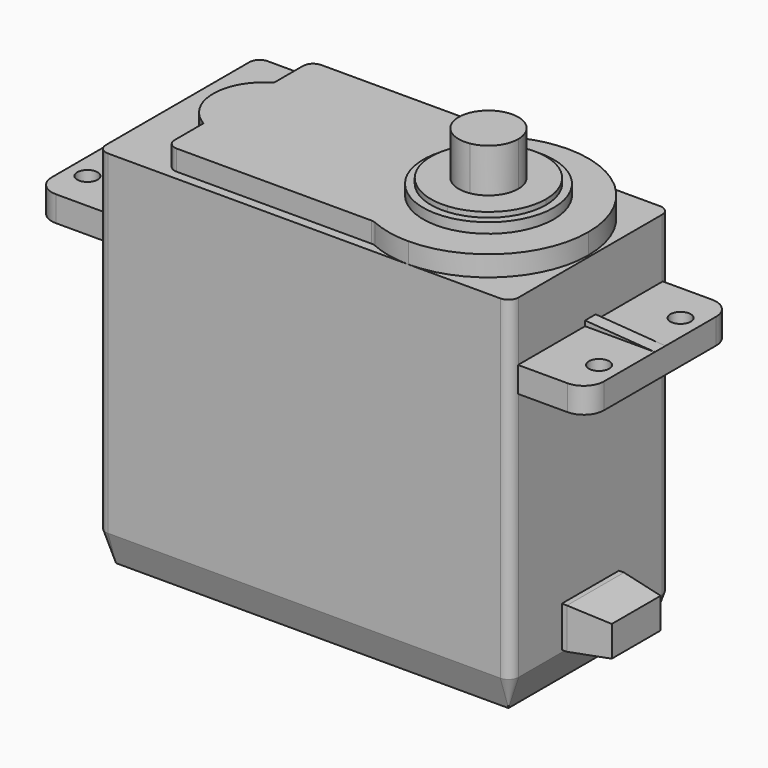
from build123d import *

# Parameters (mm, degrees)
F0_W           = 40.5
F0_H           = 2.5
F1_DEPTH       = 9.8
F0_W_2         = 6.85
F2_DEPTH       = 8.875
F0_W_3         = 4.5
F0_H_2         = 4
F3_DEPTH       = 3.5
F4_SIZE2       = 0.5
F4_SIZE        = 4
F6_DEPTH       = 2
F7_DEPTH       = 3
F8_DEPTH       = 3.5
F9_DEPTH       = 7.8
F10_DEPTH      = 0.65
F11_R          = 1
F12_DEPTH      = 5
F13_R          = 2
F14_R          = 1
F15_T4_DEPTH   = 40.8
F15_T10_DEPTH  = 40.8
F15_T16_DEPTH  = 40.8
F15_T23_DEPTH  = 40.8
F15_T29_DEPTH  = 40.8
F15_T35_DEPTH  = 40.8
F15_T41_DEPTH  = 40.8
F15_T47_DEPTH  = 40.8
F15_T54_DEPTH  = 40.8
F15_T60_DEPTH  = 40.8
F15_T66_DEPTH  = 40.8
F15_T72_DEPTH  = 40.8
F15_T78_DEPTH  = 40.8
F15_T85_DEPTH  = 40.8
F15_T91_DEPTH  = 40.8
F15_T97_DEPTH  = 40.8
F15_T103_DEPTH = 40.8
F15_T109_DEPTH = 40.8
F15_T116_DEPTH = 40.8
F15_T122_DEPTH = 40.8
F16_T1_DEPTH   = 38.5
F16_T3_DEPTH   = 17.6
F16_T6_ANGLE   = 90.0000000053
F16_T8_ANGLE   = 90.0000000053
F16_T10_ANGLE  = 90.0000000053
F16_T12_ANGLE  = 90.0000000053


# Not quite as in the source:
# - a fillet or chamfer that OpenCascade refuses, or shapes differently, is made with other operations: its cross-section is extruded or revolved along the edge and cut away or added


with BuildPart() as f1:
    # F0 (on Front) → F1 (new body, symmetric)
    with BuildSketch(Plane.XZ):
        Polygon((20.25, 17.9), (-20.25, 17.9), (-20.25, 12.6), (-20.25, 12.1), (20.25, 12.1), (20.25, 12.6), align=None)
        Polygon((20.25, 9.6), (-20.25, 9.6), (-20.25, -17.9), (20.25, -17.9), (20.25, -14.7), (20.25, -10.7), align=None)
        with Locations((0, 10.85)):
            Rectangle(F0_W, F0_H)
    extrude(amount=F1_DEPTH, both=True)

    # F0 (on Front) → F2 (join, symmetric)
    with BuildSketch(Plane.XZ):
        with Locations((23.675, 10.85)):
            Rectangle(F0_W_2, F0_H)
        with Locations((-23.675, 10.85)):
            Rectangle(F0_W_2, F0_H)
    extrude(amount=F2_DEPTH, both=True)

    # F0 (on Front) → F3 (join, symmetric)
    with BuildSketch(Plane.XZ):
        with Locations((22.5, -12.7)):
            Rectangle(F0_W_3, F0_H_2)
    extrude(amount=F3_DEPTH, both=True)

    # F4
    f4_edges = [f1.edges().sort_by_distance(p)[0] for p in [
        (24.75, 0, -10.7),
        (24.75, 3.5, -12.7),
        (24.75, -3.5, -12.7),
        (24.75, 0, -14.7),
    ]]
    chamfer(f4_edges, length=F4_SIZE, length2=F4_SIZE2)

    # F5 (on face) → F6 (join)
    with BuildSketch(Plane.XY.offset(17.9)):
        with BuildLine():
            ThreePointArc((10.2500000427, -9.8), (17.1796464707, -6.9296464405), (20.05, 0))
            ThreePointArc((20.05, 0), (17.1796464556, 6.9296464556), (10.25, 9.8))
            ThreePointArc((10.25, 9.8), (8.1210331144, 9.5659552581), (6.0937546993, 8.875))
            Line((6.0937546993, 8.875), (10.75, 8.875))
            Line((10.75, 8.875), (10.75, 6.3804388564))
            ThreePointArc((10.75, 6.3804388564), (14.9489360498, 4.3451121965), (16.65, 0))
            ThreePointArc((16.65, 0), (14.9489360498, -4.3451121965), (10.75, -6.3804388564))
            Line((10.75, -6.3804388564), (10.75, -8.875))
            Line((10.75, -8.875), (6.0937546993, -8.875))
            ThreePointArc((6.0937546993, -8.875), (8.1210331353, -9.5659552627), (10.2500000427, -9.8))
        make_face()
        with BuildLine():
            ThreePointArc((16.65, 0), (14.9489360498, 4.3451121965), (10.75, 6.3804388564))
            Line((10.75, 6.3804388564), (10.75, 5.6278326201))
            ThreePointArc((10.75, 5.6278326201), (14.4181830574, 3.8142823702), (15.9, 0))
            ThreePointArc((15.9, 0), (14.4181830574, -3.8142823702), (10.75, -5.6278326201))
            Line((10.75, -5.6278326201), (10.75, -6.3804388564))
            ThreePointArc((10.75, -6.3804388564), (14.9489360498, -4.3451121965), (16.65, 0))
        make_face()
        with BuildLine():
            ThreePointArc((15.9, 0), (14.4181830574, 3.8142823702), (10.75, 5.6278326201))
            Line((10.75, 5.6278326201), (10.75, 2.8819481258))
            ThreePointArc((10.75, 2.8819481258), (12.4880934967, 1.8832319294), (13.175, 0))
            ThreePointArc((13.175, 0), (12.4880934967, -1.8832319294), (10.75, -2.8819481258))
            Line((10.75, -2.8819481258), (10.75, -5.6278326201))
            ThreePointArc((10.75, -5.6278326201), (14.4181830574, -3.8142823702), (15.9, 0))
        make_face()
        with BuildLine():
            Line((10.75, 2.8819481258), (10.75, 5.6278326201))
            ThreePointArc((10.75, 5.6278326201), (4.6, 0), (10.75, -5.6278326201))
            Line((10.75, -5.6278326201), (10.75, -2.8819481258))
            ThreePointArc((10.75, -2.8819481258), (7.325, 0), (10.75, 2.8819481258))
        make_face()
        with BuildLine():
            Line((10.75, -2.8819481258), (10.75, 2.8819481258))
            ThreePointArc((10.75, 2.8819481258), (7.325, 0), (10.75, -2.8819481258))
        make_face()
        with BuildLine():
            ThreePointArc((13.175, 0), (12.4880934967, 1.8832319294), (10.75, 2.8819481258))
            Line((10.75, 2.8819481258), (10.75, -2.8819481258))
            ThreePointArc((10.75, -2.8819481258), (12.4880934967, -1.8832319294), (13.175, 0))
        make_face()
        with BuildLine():
            Line((10.75, 5.6278326201), (10.75, 6.3804388564))
            ThreePointArc((10.75, 6.3804388564), (3.85, 0), (10.75, -6.3804388564))
            Line((10.75, -6.3804388564), (10.75, -5.6278326201))
            ThreePointArc((10.75, -5.6278326201), (4.6, 0), (10.75, 5.6278326201))
        make_face()
        with BuildLine():
            Line((10.75, 8.875), (6.0937546993, 8.875))
            ThreePointArc((6.0937546993, 8.875), (0.45, 0), (6.0937546993, -8.875))
            Line((6.0937546993, -8.875), (10.75, -8.875))
            Line((10.75, -8.875), (10.75, -6.3804388564))
            ThreePointArc((10.75, -6.3804388564), (3.85, 0), (10.75, 6.3804388564))
            Line((10.75, 6.3804388564), (10.75, 8.875))
        make_face()
        with BuildLine():
            ThreePointArc((6.0937546993, -8.875), (0.45, 0), (6.0937546993, 8.875))
            Line((6.0937546993, 8.875), (-14.25, 8.875))
            Line((-14.25, 8.875), (-14.25, 4.3301270189))
            ThreePointArc((-14.25, 4.3301270189), (-9.25, 4.3301270189), (-6.75, 0))
            ThreePointArc((-6.75, 0), (-9.25, -4.3301270189), (-14.25, -4.3301270189))
            Line((-14.25, -4.3301270189), (-14.25, -8.875))
            Line((-14.25, -8.875), (6.0937546993, -8.875))
        make_face()
        with BuildLine():
            ThreePointArc((-6.75, 0), (-9.25, 4.3301270189), (-14.25, 4.3301270189))
            Line((-14.25, 4.3301270189), (-14.25, -4.3301270189))
            ThreePointArc((-14.25, -4.3301270189), (-9.25, -4.3301270189), (-6.75, 0))
        make_face()
        with BuildLine():
            Line((-14.25, -4.3301270189), (-14.25, 4.3301270189))
            ThreePointArc((-14.25, 4.3301270189), (-16.75, 0), (-14.25, -4.3301270189))
        make_face()
    extrude(amount=F6_DEPTH)

    # F5 (on face) → F7 (join)
    with BuildSketch(Plane.XY.offset(17.9)):
        with BuildLine():
            Line((10.75, 2.8819481258), (10.75, 5.6278326201))
            ThreePointArc((10.75, 5.6278326201), (4.6, 0), (10.75, -5.6278326201))
            Line((10.75, -5.6278326201), (10.75, -2.8819481258))
            ThreePointArc((10.75, -2.8819481258), (7.325, 0), (10.75, 2.8819481258))
        make_face()
        with BuildLine():
            Line((10.75, -2.8819481258), (10.75, 2.8819481258))
            ThreePointArc((10.75, 2.8819481258), (7.325, 0), (10.75, -2.8819481258))
        make_face()
        with BuildLine():
            ThreePointArc((13.175, 0), (12.4880934967, 1.8832319294), (10.75, 2.8819481258))
            Line((10.75, 2.8819481258), (10.75, -2.8819481258))
            ThreePointArc((10.75, -2.8819481258), (12.4880934967, -1.8832319294), (13.175, 0))
        make_face()
        with BuildLine():
            ThreePointArc((15.9, 0), (14.4181830574, 3.8142823702), (10.75, 5.6278326201))
            Line((10.75, 5.6278326201), (10.75, 2.8819481258))
            ThreePointArc((10.75, 2.8819481258), (12.4880934967, 1.8832319294), (13.175, 0))
            ThreePointArc((13.175, 0), (12.4880934967, -1.8832319294), (10.75, -2.8819481258))
            Line((10.75, -2.8819481258), (10.75, -5.6278326201))
            ThreePointArc((10.75, -5.6278326201), (14.4181830574, -3.8142823702), (15.9, 0))
        make_face()
        with BuildLine():
            ThreePointArc((16.65, 0), (14.9489360498, 4.3451121965), (10.75, 6.3804388564))
            Line((10.75, 6.3804388564), (10.75, 5.6278326201))
            ThreePointArc((10.75, 5.6278326201), (14.4181830574, 3.8142823702), (15.9, 0))
            ThreePointArc((15.9, 0), (14.4181830574, -3.8142823702), (10.75, -5.6278326201))
            Line((10.75, -5.6278326201), (10.75, -6.3804388564))
            ThreePointArc((10.75, -6.3804388564), (14.9489360498, -4.3451121965), (16.65, 0))
        make_face()
        with BuildLine():
            Line((10.75, 5.6278326201), (10.75, 6.3804388564))
            ThreePointArc((10.75, 6.3804388564), (3.85, 0), (10.75, -6.3804388564))
            Line((10.75, -6.3804388564), (10.75, -5.6278326201))
            ThreePointArc((10.75, -5.6278326201), (4.6, 0), (10.75, 5.6278326201))
        make_face()
    extrude(amount=F7_DEPTH)

    # F5 (on face) → F8 (join)
    with BuildSketch(Plane.XY.offset(17.9)):
        with BuildLine():
            ThreePointArc((13.175, 0), (12.4880934967, 1.8832319294), (10.75, 2.8819481258))
            Line((10.75, 2.8819481258), (10.75, -2.8819481258))
            ThreePointArc((10.75, -2.8819481258), (12.4880934967, -1.8832319294), (13.175, 0))
        make_face()
        with BuildLine():
            Line((10.75, -2.8819481258), (10.75, 2.8819481258))
            ThreePointArc((10.75, 2.8819481258), (7.325, 0), (10.75, -2.8819481258))
        make_face()
        with BuildLine():
            Line((10.75, 2.8819481258), (10.75, 5.6278326201))
            ThreePointArc((10.75, 5.6278326201), (4.6, 0), (10.75, -5.6278326201))
            Line((10.75, -5.6278326201), (10.75, -2.8819481258))
            ThreePointArc((10.75, -2.8819481258), (7.325, 0), (10.75, 2.8819481258))
        make_face()
        with BuildLine():
            ThreePointArc((15.9, 0), (14.4181830574, 3.8142823702), (10.75, 5.6278326201))
            Line((10.75, 5.6278326201), (10.75, 2.8819481258))
            ThreePointArc((10.75, 2.8819481258), (12.4880934967, 1.8832319294), (13.175, 0))
            ThreePointArc((13.175, 0), (12.4880934967, -1.8832319294), (10.75, -2.8819481258))
            Line((10.75, -2.8819481258), (10.75, -5.6278326201))
            ThreePointArc((10.75, -5.6278326201), (14.4181830574, -3.8142823702), (15.9, 0))
        make_face()
    extrude(amount=F8_DEPTH)

    # F5 (on face) → F9 (join)
    with BuildSketch(Plane.XY.offset(17.9)):
        with BuildLine():
            Line((10.75, -2.8819481258), (10.75, 2.8819481258))
            ThreePointArc((10.75, 2.8819481258), (7.325, 0), (10.75, -2.8819481258))
        make_face()
        with BuildLine():
            ThreePointArc((13.175, 0), (12.4880934967, 1.8832319294), (10.75, 2.8819481258))
            Line((10.75, 2.8819481258), (10.75, -2.8819481258))
            ThreePointArc((10.75, -2.8819481258), (12.4880934967, -1.8832319294), (13.175, 0))
        make_face()
    extrude(amount=F9_DEPTH)

    # F0 (on Front) → F10 (join, symmetric)
    with BuildSketch(Plane.XZ):
        Polygon((27.1, 12.1), (20.25, 12.6), (20.25, 12.1), align=None)
        Polygon((-20.25, 12.1), (-20.25, 12.6), (-27.1, 12.1), align=None)
    extrude(amount=F10_DEPTH, both=True)

    # F11 (on face) → F12 (cut)
    with BuildSketch(Plane.XY.offset(12.1)):
        with Locations((-25.1, 5)):
            Circle(F11_R)
        with Locations((-25.1, -5)):
            Circle(F11_R)
        with Locations((25.1, 5)):
            Circle(F11_R)
        with Locations((25.1, -5)):
            Circle(F11_R)
    extrude(amount=-F12_DEPTH, mode=Mode.SUBTRACT)

    # F13
    f13_edges = [f1.edges().sort_by_distance(p)[0] for p in [
        (27.1, -8.875, 10.85),
        (27.1, 8.875, 10.85),
        (-27.1, -8.875, 10.85),
        (-27.1, 8.875, 10.85),
    ]]
    fillet(f13_edges, radius=F13_R)

    # F14
    f14_edges = [f1.edges().sort_by_distance(p)[0] for p in [
        (-14.25, -8.875, 18.9),
        (-14.25, 8.875, 18.9),
        (6.093755, 8.875, 18.9),
        (6.093755, -8.875, 18.9),
    ]]
    fillet(f14_edges, radius=F14_R)

    # F15: fillet of radius 1 on 4 edges, made by hand


with BuildPart() as f15_tool2:
    # F15_s3 → F15_t4 (new body)
    with BuildSketch(Plane.XY.offset(-20.4)):
        with BuildLine():
            ThreePointArc((19.25, -9.8), (19.9571067812, -9.5071067812), (20.25, -8.8))
            Line((20.25, -8.8), (20.25, -9.8))
            Line((20.25, -9.8), (19.25, -9.8))
        make_face()
    extrude(amount=F15_T4_DEPTH)

    split(bisect_by=Plane.XZ.offset(8.875), keep=Keep.TOP)

    split(bisect_by=Plane.XY.offset(9.6), keep=Keep.BOTTOM)


with BuildPart() as f1_1:
    add(f1.part)

    # F15_t1: cut F15_tool2
    add(f15_tool2.part, mode=Mode.SUBTRACT)


with BuildPart() as f15_tool8:
    # F15_s9 → F15_t10 (new body)
    with BuildSketch(Plane.XY.offset(-20.4)):
        with BuildLine():
            ThreePointArc((19.25, -9.8), (19.9571067812, -9.5071067812), (20.25, -8.8))
            Line((20.25, -8.8), (20.25, -9.8))
            Line((20.25, -9.8), (19.25, -9.8))
        make_face()
    extrude(amount=F15_T10_DEPTH)

    split(bisect_by=Plane.XZ.offset(8.875), keep=Keep.BOTTOM)

    split(bisect_by=Plane.XY.offset(9.6), keep=Keep.BOTTOM)


with BuildPart() as f1_2:
    add(f1_1.part)

    # F15_t7: cut F15_tool8
    add(f15_tool8.part, mode=Mode.SUBTRACT)


with BuildPart() as f15_tool14:
    # F15_s15 → F15_t16 (new body)
    with BuildSketch(Plane.XY.offset(-20.4)):
        with BuildLine():
            ThreePointArc((19.25, -9.8), (19.9571067812, -9.5071067812), (20.25, -8.8))
            Line((20.25, -8.8), (20.25, -9.8))
            Line((20.25, -9.8), (19.25, -9.8))
        make_face()
    extrude(amount=F15_T16_DEPTH)

    split(bisect_by=Plane.XY.offset(12.1), keep=Keep.BOTTOM)

    split(bisect_by=Plane.XZ.offset(8.875), keep=Keep.TOP)

    split(bisect_by=Plane.XY.offset(9.6), keep=Keep.TOP)


with BuildPart() as f1_3:
    add(f1_2.part)

    # F15_t13: cut F15_tool14
    add(f15_tool14.part, mode=Mode.SUBTRACT)


with BuildPart() as f15_tool21:
    # F15_s22 → F15_t23 (new body)
    with BuildSketch(Plane.XY.offset(-20.4)):
        with BuildLine():
            ThreePointArc((19.25, -9.8), (19.9571067812, -9.5071067812), (20.25, -8.8))
            Line((20.25, -8.8), (20.25, -9.8))
            Line((20.25, -9.8), (19.25, -9.8))
        make_face()
    extrude(amount=F15_T23_DEPTH)

    split(bisect_by=Plane.XY.offset(12.1), keep=Keep.TOP)

    split(bisect_by=Plane.XZ.offset(8.875), keep=Keep.TOP)


with BuildPart() as f1_4:
    add(f1_3.part)

    # F15_t20: cut F15_tool21
    add(f15_tool21.part, mode=Mode.SUBTRACT)


with BuildPart() as f15_tool27:
    # F15_s28 → F15_t29 (new body)
    with BuildSketch(Plane.XY.offset(-20.4)):
        with BuildLine():
            ThreePointArc((19.25, -9.8), (19.9571067812, -9.5071067812), (20.25, -8.8))
            Line((20.25, -8.8), (20.25, -9.8))
            Line((20.25, -9.8), (19.25, -9.8))
        make_face()
    extrude(amount=F15_T29_DEPTH)

    split(bisect_by=Plane.XY.offset(12.1), keep=Keep.TOP)

    split(bisect_by=Plane.XZ.offset(8.875), keep=Keep.BOTTOM)


with BuildPart() as f1_5:
    add(f1_4.part)

    # F15_t26: cut F15_tool27
    add(f15_tool27.part, mode=Mode.SUBTRACT)


with BuildPart() as f15_tool33:
    # F15_s34 → F15_t35 (new body)
    with BuildSketch(Plane.XY.offset(20.4)):
        with BuildLine():
            ThreePointArc((-20.25, -8.8), (-19.9571067812, -9.5071067812), (-19.25, -9.8))
            Line((-19.25, -9.8), (-20.25, -9.8))
            Line((-20.25, -9.8), (-20.25, -8.8))
        make_face()
    extrude(amount=-F15_T35_DEPTH)

    split(bisect_by=Plane.XZ.offset(8.875), keep=Keep.BOTTOM)

    split(bisect_by=Plane.XY.offset(12.1), keep=Keep.TOP)


with BuildPart() as f1_6:
    add(f1_5.part)

    # F15_t32: cut F15_tool33
    add(f15_tool33.part, mode=Mode.SUBTRACT)


with BuildPart() as f15_tool39:
    # F15_s40 → F15_t41 (new body)
    with BuildSketch(Plane.XY.offset(20.4)):
        with BuildLine():
            ThreePointArc((-20.25, -8.8), (-19.9571067812, -9.5071067812), (-19.25, -9.8))
            Line((-19.25, -9.8), (-20.25, -9.8))
            Line((-20.25, -9.8), (-20.25, -8.8))
        make_face()
    extrude(amount=-F15_T41_DEPTH)

    split(bisect_by=Plane.XZ.offset(8.875), keep=Keep.TOP)

    split(bisect_by=Plane.XY.offset(12.1), keep=Keep.TOP)


with BuildPart() as f1_7:
    add(f1_6.part)

    # F15_t38: cut F15_tool39
    add(f15_tool39.part, mode=Mode.SUBTRACT)


with BuildPart() as f15_tool45:
    # F15_s46 → F15_t47 (new body)
    with BuildSketch(Plane.XY.offset(20.4)):
        with BuildLine():
            ThreePointArc((-20.25, -8.8), (-19.9571067812, -9.5071067812), (-19.25, -9.8))
            Line((-19.25, -9.8), (-20.25, -9.8))
            Line((-20.25, -9.8), (-20.25, -8.8))
        make_face()
    extrude(amount=-F15_T47_DEPTH)

    split(bisect_by=Plane.XZ.offset(8.875), keep=Keep.TOP)

    split(bisect_by=Plane.XY.offset(12.1), keep=Keep.BOTTOM)

    split(bisect_by=Plane.XY.offset(9.6), keep=Keep.TOP)


with BuildPart() as f1_8:
    add(f1_7.part)

    # F15_t44: cut F15_tool45
    add(f15_tool45.part, mode=Mode.SUBTRACT)


with BuildPart() as f15_tool52:
    # F15_s53 → F15_t54 (new body)
    with BuildSketch(Plane.XY.offset(20.4)):
        with BuildLine():
            ThreePointArc((-20.25, -8.8), (-19.9571067812, -9.5071067812), (-19.25, -9.8))
            Line((-19.25, -9.8), (-20.25, -9.8))
            Line((-20.25, -9.8), (-20.25, -8.8))
        make_face()
    extrude(amount=-F15_T54_DEPTH)

    split(bisect_by=Plane.XZ.offset(8.875), keep=Keep.BOTTOM)

    split(bisect_by=Plane.XY.offset(9.6), keep=Keep.BOTTOM)


with BuildPart() as f1_9:
    add(f1_8.part)

    # F15_t51: cut F15_tool52
    add(f15_tool52.part, mode=Mode.SUBTRACT)


with BuildPart() as f15_tool58:
    # F15_s59 → F15_t60 (new body)
    with BuildSketch(Plane.XY.offset(20.4)):
        with BuildLine():
            ThreePointArc((-20.25, -8.8), (-19.9571067812, -9.5071067812), (-19.25, -9.8))
            Line((-19.25, -9.8), (-20.25, -9.8))
            Line((-20.25, -9.8), (-20.25, -8.8))
        make_face()
    extrude(amount=-F15_T60_DEPTH)

    split(bisect_by=Plane.XZ.offset(8.875), keep=Keep.TOP)

    split(bisect_by=Plane.XY.offset(9.6), keep=Keep.BOTTOM)


with BuildPart() as f1_10:
    add(f1_9.part)

    # F15_t57: cut F15_tool58
    add(f15_tool58.part, mode=Mode.SUBTRACT)


with BuildPart() as f15_tool64:
    # F15_s65 → F15_t66 (new body)
    with BuildSketch(Plane.XY.offset(20.4)):
        with BuildLine():
            ThreePointArc((-19.25, 9.8), (-19.9571067812, 9.5071067812), (-20.25, 8.8))
            Line((-20.25, 8.8), (-20.25, 9.8))
            Line((-20.25, 9.8), (-19.25, 9.8))
        make_face()
    extrude(amount=-F15_T66_DEPTH)

    split(bisect_by=Plane.XY.offset(12.1), keep=Keep.TOP)

    split(bisect_by=Plane.XZ.offset(-8.875), keep=Keep.BOTTOM)


with BuildPart() as f1_11:
    add(f1_10.part)

    # F15_t63: cut F15_tool64
    add(f15_tool64.part, mode=Mode.SUBTRACT)


with BuildPart() as f15_tool70:
    # F15_s71 → F15_t72 (new body)
    with BuildSketch(Plane.XY.offset(20.4)):
        with BuildLine():
            ThreePointArc((-19.25, 9.8), (-19.9571067812, 9.5071067812), (-20.25, 8.8))
            Line((-20.25, 8.8), (-20.25, 9.8))
            Line((-20.25, 9.8), (-19.25, 9.8))
        make_face()
    extrude(amount=-F15_T72_DEPTH)

    split(bisect_by=Plane.XY.offset(12.1), keep=Keep.TOP)

    split(bisect_by=Plane.XZ.offset(-8.875), keep=Keep.TOP)


with BuildPart() as f1_12:
    add(f1_11.part)

    # F15_t69: cut F15_tool70
    add(f15_tool70.part, mode=Mode.SUBTRACT)


with BuildPart() as f15_tool76:
    # F15_s77 → F15_t78 (new body)
    with BuildSketch(Plane.XY.offset(20.4)):
        with BuildLine():
            ThreePointArc((-19.25, 9.8), (-19.9571067812, 9.5071067812), (-20.25, 8.8))
            Line((-20.25, 8.8), (-20.25, 9.8))
            Line((-20.25, 9.8), (-19.25, 9.8))
        make_face()
    extrude(amount=-F15_T78_DEPTH)

    split(bisect_by=Plane.XY.offset(12.1), keep=Keep.BOTTOM)

    split(bisect_by=Plane.XZ.offset(-8.875), keep=Keep.BOTTOM)

    split(bisect_by=Plane.XY.offset(9.6), keep=Keep.TOP)


with BuildPart() as f1_13:
    add(f1_12.part)

    # F15_t75: cut F15_tool76
    add(f15_tool76.part, mode=Mode.SUBTRACT)


with BuildPart() as f15_tool83:
    # F15_s84 → F15_t85 (new body)
    with BuildSketch(Plane.XY.offset(20.4)):
        with BuildLine():
            ThreePointArc((-19.25, 9.8), (-19.9571067812, 9.5071067812), (-20.25, 8.8))
            Line((-20.25, 8.8), (-20.25, 9.8))
            Line((-20.25, 9.8), (-19.25, 9.8))
        make_face()
    extrude(amount=-F15_T85_DEPTH)

    split(bisect_by=Plane.XZ.offset(-8.875), keep=Keep.BOTTOM)

    split(bisect_by=Plane.XY.offset(9.6), keep=Keep.BOTTOM)


with BuildPart() as f1_14:
    add(f1_13.part)

    # F15_t82: cut F15_tool83
    add(f15_tool83.part, mode=Mode.SUBTRACT)


with BuildPart() as f15_tool89:
    # F15_s90 → F15_t91 (new body)
    with BuildSketch(Plane.XY.offset(20.4)):
        with BuildLine():
            ThreePointArc((-19.25, 9.8), (-19.9571067812, 9.5071067812), (-20.25, 8.8))
            Line((-20.25, 8.8), (-20.25, 9.8))
            Line((-20.25, 9.8), (-19.25, 9.8))
        make_face()
    extrude(amount=-F15_T91_DEPTH)

    split(bisect_by=Plane.XZ.offset(-8.875), keep=Keep.TOP)

    split(bisect_by=Plane.XY.offset(9.6), keep=Keep.BOTTOM)


with BuildPart() as f1_15:
    add(f1_14.part)

    # F15_t88: cut F15_tool89
    add(f15_tool89.part, mode=Mode.SUBTRACT)


with BuildPart() as f15_tool95:
    # F15_s96 → F15_t97 (new body)
    with BuildSketch(Plane.XY.offset(-20.4)):
        with BuildLine():
            ThreePointArc((19.25, 9.8), (19.9571067812, 9.5071067812), (20.25, 8.8))
            Line((20.25, 8.8), (20.25, 9.8))
            Line((20.25, 9.8), (19.25, 9.8))
        make_face()
    extrude(amount=F15_T97_DEPTH)

    split(bisect_by=Plane.XY.offset(9.6), keep=Keep.BOTTOM)

    split(bisect_by=Plane.XZ.offset(-8.875), keep=Keep.BOTTOM)


with BuildPart() as f1_16:
    add(f1_15.part)

    # F15_t94: cut F15_tool95
    add(f15_tool95.part, mode=Mode.SUBTRACT)


with BuildPart() as f15_tool101:
    # F15_s102 → F15_t103 (new body)
    with BuildSketch(Plane.XY.offset(-20.4)):
        with BuildLine():
            ThreePointArc((19.25, 9.8), (19.9571067812, 9.5071067812), (20.25, 8.8))
            Line((20.25, 8.8), (20.25, 9.8))
            Line((20.25, 9.8), (19.25, 9.8))
        make_face()
    extrude(amount=F15_T103_DEPTH)

    split(bisect_by=Plane.XY.offset(9.6), keep=Keep.BOTTOM)

    split(bisect_by=Plane.XZ.offset(-8.875), keep=Keep.TOP)


with BuildPart() as f1_17:
    add(f1_16.part)

    # F15_t100: cut F15_tool101
    add(f15_tool101.part, mode=Mode.SUBTRACT)


with BuildPart() as f15_tool107:
    # F15_s108 → F15_t109 (new body)
    with BuildSketch(Plane.XY.offset(-20.4)):
        with BuildLine():
            ThreePointArc((19.25, 9.8), (19.9571067812, 9.5071067812), (20.25, 8.8))
            Line((20.25, 8.8), (20.25, 9.8))
            Line((20.25, 9.8), (19.25, 9.8))
        make_face()
    extrude(amount=F15_T109_DEPTH)

    split(bisect_by=Plane.XY.offset(12.1), keep=Keep.BOTTOM)

    split(bisect_by=Plane.XY.offset(9.6), keep=Keep.TOP)

    split(bisect_by=Plane.XZ.offset(-8.875), keep=Keep.BOTTOM)


with BuildPart() as f1_18:
    add(f1_17.part)

    # F15_t106: cut F15_tool107
    add(f15_tool107.part, mode=Mode.SUBTRACT)


with BuildPart() as f15_tool114:
    # F15_s115 → F15_t116 (new body)
    with BuildSketch(Plane.XY.offset(-20.4)):
        with BuildLine():
            ThreePointArc((19.25, 9.8), (19.9571067812, 9.5071067812), (20.25, 8.8))
            Line((20.25, 8.8), (20.25, 9.8))
            Line((20.25, 9.8), (19.25, 9.8))
        make_face()
    extrude(amount=F15_T116_DEPTH)

    split(bisect_by=Plane.XY.offset(12.1), keep=Keep.TOP)

    split(bisect_by=Plane.XZ.offset(-8.875), keep=Keep.BOTTOM)


with BuildPart() as f1_19:
    add(f1_18.part)

    # F15_t113: cut F15_tool114
    add(f15_tool114.part, mode=Mode.SUBTRACT)


with BuildPart() as f15_tool120:
    # F15_s121 → F15_t122 (new body)
    with BuildSketch(Plane.XY.offset(-20.4)):
        with BuildLine():
            ThreePointArc((19.25, 9.8), (19.9571067812, 9.5071067812), (20.25, 8.8))
            Line((20.25, 8.8), (20.25, 9.8))
            Line((20.25, 9.8), (19.25, 9.8))
        make_face()
    extrude(amount=F15_T122_DEPTH)

    split(bisect_by=Plane.XY.offset(12.1), keep=Keep.TOP)

    split(bisect_by=Plane.XZ.offset(-8.875), keep=Keep.TOP)


with BuildPart() as f1_20:
    add(f1_19.part)

    # F15_t119: cut F15_tool120
    add(f15_tool120.part, mode=Mode.SUBTRACT)

    # F16: chamfer of 3 x 1 on 8 edges, made by hand

    # F16_s2 → F16_t1 (cut)
    with BuildSketch(Plane.YZ.offset(-19.25)):
        Polygon((-9.8, -14.9), (-8.8, -17.9), (-9.8, -17.9), align=None)
        Polygon((8.8, -17.9), (9.8, -14.9), (9.8, -17.9), align=None)
    extrude(amount=F16_T1_DEPTH, mode=Mode.SUBTRACT)

    # F16_s4 → F16_t3 (cut)
    with BuildSketch(Plane.XZ.offset(-8.8)):
        Polygon((20.25, -14.9), (19.25, -17.9), (20.25, -17.9), align=None)
        Polygon((-19.25, -17.9), (-20.25, -14.9), (-20.25, -17.9), align=None)
    extrude(amount=F16_T3_DEPTH, mode=Mode.SUBTRACT)

    # F16_s5 → F16_t6 (revolve, cut)
    with BuildSketch(Plane.XZ.offset(-8.8)):
        Polygon((20.25, -14.9), (19.25, -17.9), (20.25, -17.9), align=None)
    revolve(axis=Axis((19.25, 8.8, -17.9), (0, 0, 1)), revolution_arc=F16_T6_ANGLE, mode=Mode.SUBTRACT)

    # F16_s7 → F16_t8 (revolve, cut)
    with BuildSketch(Plane.XZ.offset(8.8)):
        Polygon((20.25, -14.9), (19.25, -17.9), (20.25, -17.9), align=None)
    revolve(axis=Axis((19.25, -8.8, -17.9), (0, 0, -1)), revolution_arc=F16_T8_ANGLE, mode=Mode.SUBTRACT)

    # F16_s9 → F16_t10 (revolve, cut)
    with BuildSketch(Plane.YZ.offset(-19.25)):
        Polygon((8.8, -17.9), (9.8, -14.9), (9.8, -17.9), align=None)
    revolve(axis=Axis((-19.25, 8.8, -17.9), (0, 0, 1)), revolution_arc=F16_T10_ANGLE, mode=Mode.SUBTRACT)

    # F16_s11 → F16_t12 (revolve, cut)
    with BuildSketch(Plane.XZ.offset(8.8)):
        Polygon((-19.25, -17.9), (-20.25, -14.9), (-20.25, -17.9), align=None)
    revolve(axis=Axis((-19.25, -8.8, -17.9), (0, 0, 1)), revolution_arc=F16_T12_ANGLE, mode=Mode.SUBTRACT)


solid = f1_20.part
